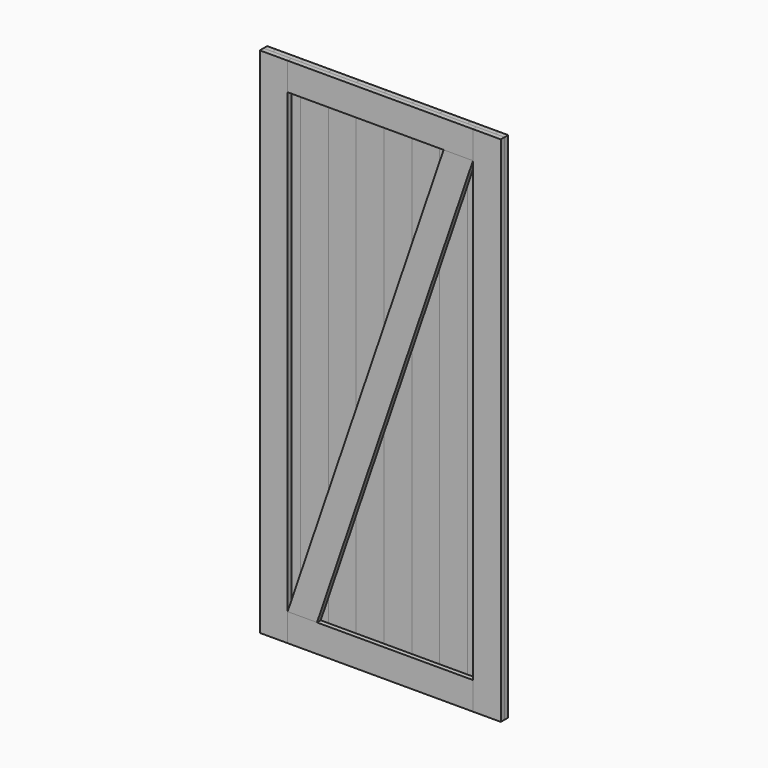
from build123d import *

# Parameters (mm, degrees)
F0_W            = 114.3
F0_H            = 19.05
F1_DEPTH        = 2108.2
F1_COPIES_COUNT = 4
F1_COPIES_PITCH = 228.6
F5_W            = 38.1
F5_H            = 19.05
F6_DEPTH        = 2108.2
F10_W           = 762
F10_H           = 114.3
F11_DEPTH       = 19.05
F14_DEPTH       = 19.05


# Not quite as in the source:
# - a feature of the source that left no trace in its solid (it failed there, or was rolled back) is left out
# - a pattern or mirror of a feature is missing from the dataset's text; its kind, count and spacing are read off the source's solid


with BuildPart() as f1:
    # F0 (on Top) → F1 (new body)
    with BuildSketch(Plane.XY):
        with Locations((57.15, 9.525)):
            Rectangle(F0_W, F0_H)
    extrude(amount=F1_DEPTH)


with BuildPart() as f1_copies_1:
    # F1_copies: instance of F1
    add(f1.part.moved(Location(Vector(1, 0, 0) * (1 * F1_COPIES_PITCH))))


with BuildPart() as f1_copies_2:
    # F1_copies: instance of F1
    add(f1.part.moved(Location(Vector(1, 0, 0) * (2 * F1_COPIES_PITCH))))


with BuildPart() as f1_copies_3:
    # F1_copies: instance of F1
    add(f1.part.moved(Location(Vector(1, 0, 0) * (3 * F1_COPIES_PITCH))))


with BuildPart() as f1_copies1_1:
    # F1_copies1: instance of F1
    add(f1.part.mirror(Plane(origin=(342.9, 0, 0), x_dir=(0, 0, 1), z_dir=(1, 0, 0))))


with BuildPart() as f1_copies2_1:
    # F1_copies2: instance of F1
    add(f1.part.mirror(Plane(origin=(228.6, 0, 0), x_dir=(0, 0, 1), z_dir=(1, 0, 0))))


with BuildPart() as f1_copies3_1:
    # F1_copies3: instance of F1
    add(f1.part.mirror(Plane(origin=(457.2, 0, 0), x_dir=(0, 0, 1), z_dir=(1, 0, 0))))


with BuildPart() as f2_1:
    # F2: copy of F1
    add(f1.part.moved(Location((114.3, 0, 0))))


with BuildPart() as f6:
    # F5 (on Top) → F6 (new body)
    with BuildSketch(Plane.XY):
        with Locations((-19.05, 9.525)):
            Rectangle(F5_W, F5_H)
    extrude(amount=F6_DEPTH)


with BuildPart() as f7_1:
    # F7: copy of F6
    add(f6.part.moved(Location((952.5, 0, 0))))


with BuildPart() as f8_1:
    # F8: copy of F1
    add(f1.part.moved(Location((-38.1, -19.05, 0))))


with BuildPart() as f9_1:
    # F9: copy of F8_1
    add(f8_1.part.moved(Location((876.3, 0, 0))))


with BuildPart() as f11:
    # F10 (on face) → F11 (new body)
    with BuildSketch(Plane.XZ):
        with Locations((457.2, 2051.05)):
            Rectangle(F10_W, F10_H)
    extrude(amount=F11_DEPTH)


with BuildPart() as f12_1:
    # F12: copy of F11
    add(f11.part.moved(Location((0, 0, -1993.9))))


with BuildPart() as f14:
    # F13 (on face) → F14 (new body)
    with BuildSketch(Plane.XZ):
        Polygon((717.4315957213, 1993.9), (76.2, 114.3), (196.9684042787, 114.3), (838.2, 1993.9), align=None)
    extrude(amount=F14_DEPTH)


solid = Compound([f1.part, f1_copies_1.part, f1_copies_2.part, f1_copies_3.part, f1_copies1_1.part, f1_copies2_1.part, f1_copies3_1.part, f2_1.part, f6.part, f7_1.part, f8_1.part, f9_1.part, f11.part, f12_1.part, f14.part])
